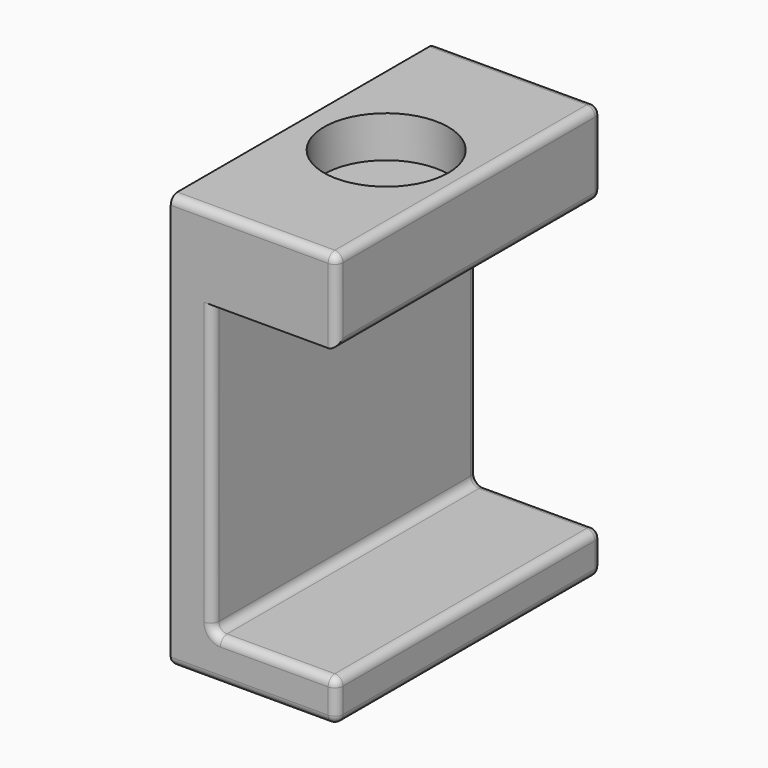
from build123d import *

# Parameters (mm, degrees)
F1_DEPTH = 40
F2_R     = 7.5
F3_DEPTH = 5
F4_R     = 1


with BuildPart() as f1:
    # F0 (on Front) → F1 (new body)
    with BuildSketch(Plane.XZ):
        Polygon((-12.1263185228, 49.3127419949), (-32.1263185228, 49.3127419949), (-32.1263185228, -0.6872580051), (-12.1263185228, -0.6872580051), (-12.1263185228, 4.3127419949), (-27.1263185228, 4.3127419949), (-27.1263185228, 39.3127419949), (-12.1263185228, 39.3127419949), align=None)
    extrude(amount=F1_DEPTH)

    # F2 (on face) → F3 (cut)
    with BuildSketch(Plane.XY.offset(49.3127419949)):
        with Locations((-22.1263185228, -20)):
            Circle(F2_R)
    extrude(amount=-F3_DEPTH, mode=Mode.SUBTRACT)

    # F4
    f4_edges = [f1.edges().sort_by_distance(p)[0] for p in [
        (-22.126319, -40, 49.312742),
        (-12.126319, -20, 39.312742),
        (-12.126319, -20, 49.312742),
        (-12.126319, 0, 44.312742),
        (-12.126319, -40, 44.312742),
        (-22.126319, 0, 49.312742),
        (-32.126319, 0, 24.312742),
        (-22.126319, 0, -0.687258),
        (-12.126319, 0, 1.812742),
        (-19.626319, 0, 4.312742),
        (-27.126319, 0, 21.812742),
        (-19.626319, 0, 39.312742),
        (-12.126319, -20, 4.312742),
        (-27.126319, -20, 4.312742),
        (-19.626319, -40, 4.312742),
        (-32.126319, -20, -0.687258),
        (-12.126319, -20, -0.687258),
        (-22.126319, -40, -0.687258),
        (-12.126319, -40, 1.812742),
        (-27.126319, -40, 21.812742),
    ]]
    fillet(f4_edges, radius=F4_R)


solid = f1.part
